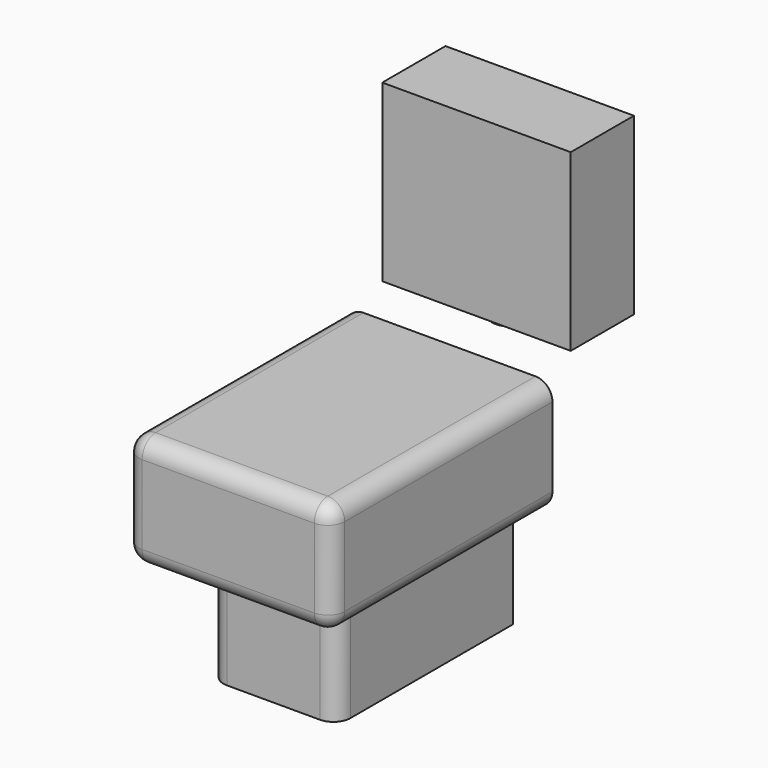
from build123d import *

# Parameters (mm, degrees)
F0_W      = 225
F0_H      = 390
F1_DEPTH  = 200
F2_W      = 182.5
F2_H      = 295
F2_H_2    = 195
F3_DEPTH  = 200
F4_R      = 30
F5_R      = 51
F6_DEPTH  = 100
F5_R_2    = 27.5
F7_DEPTH  = 60
F10_DEPTH = 310
F11_R     = 27.5
F12_DEPTH = 30


with BuildPart() as f1:
    # F0 (on Top) → F1 (new body)
    with BuildSketch(Plane.XY):
        with Locations((112.5, -195)):
            Rectangle(F0_W, F0_H)
    extrude(amount=F1_DEPTH)

    # F2 (on face) → F3 (join)
    with BuildSketch(Plane.XY.offset(200)):
        with Locations((21.25, -342.5)):
            Rectangle(F2_W, F2_H)
        with Locations((21.25, -97.5)):
            Rectangle(F2_W, F2_H_2)
        Polygon((112.5, 0), (112.5, -195), (112.5, -490), (295, -490), (295, 0), align=None)
    extrude(amount=F3_DEPTH)

    # F4
    f4_edges = [f1.edges().sort_by_distance(p)[0] for p in [
        (225, -390, 100),
        (112.5, -390, 200),
        (0, -390, 100),
        (295, -245, 200),
        (112.5, -490, 200),
        (-70, -245, 200),
        (-70, -490, 300),
        (295, -490, 300),
        (112.5, -490, 400),
        (-70, -245, 400),
        (295, -245, 400),
        (0, -195, 200),
        (225, -195, 200),
    ]]
    fillet(f4_edges, radius=F4_R)

    # F5 (on face) → F6 (join)
    with BuildSketch(Plane(origin=(0, 0, 0), x_dir=(-1, 0, 0), z_dir=(0, 1, 0))):
        with Locations((-112.5, 180)):
            Circle(F5_R)
    extrude(amount=F6_DEPTH)

    # F5 (on face) → F7 (join)
    with BuildSketch(Plane(origin=(0, 0, 0), x_dir=(-1, 0, 0), z_dir=(0, 1, 0))):
        with Locations((-112.5, 330)):
            Circle(F5_R_2)
    extrude(amount=F7_DEPTH)


with BuildPart() as f10:
    # F9 (on offset) → F10 (new body)
    with BuildSketch(Plane.XY.offset(420)):
        Polygon((-54.5, 60), (112.5, 60), (279.5, 60), (279.5, 200), (-54.5, 200), align=None)
    extrude(amount=F10_DEPTH)

    # F11 (on face) → F12 (join)
    with BuildSketch(Plane(origin=(0, 0, 420), x_dir=(1, 0, 0), z_dir=(0, 0, -1))):
        with Locations((112.5, -130)):
            Circle(F11_R)
    extrude(amount=F12_DEPTH)


solid = Compound([f1.part, f10.part])
